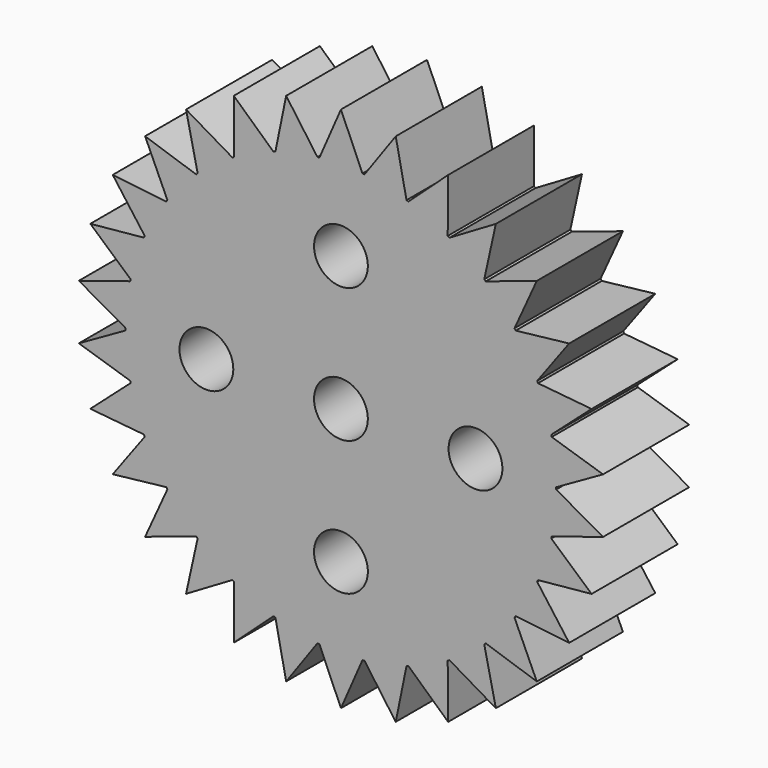
from build123d import *

# Parameters (mm, degrees)
F0_R            = 12.7
F1_DEPTH        = 3.175
F3_DEPTH        = 6.35
F3_COPIES_COUNT = 30
F4_R            = 1.5875
F5_DEPTH        = 6.35
F6_R            = 1.5875
F7_DEPTH        = 6.35
F7_COPIES_COUNT = 4


# Not quite as in the source:
# - a pattern or mirror of a feature is missing from the dataset's text; its kind, count and spacing are read off the source's solid
# - a feature names something its author has since deleted; it is built from what else it names


with BuildPart() as f1:
    # F0 (on Front) → F1 (new body, symmetric)
    with BuildSketch(Plane.XZ):
        Circle(F0_R)
    extrude(amount=F1_DEPTH, both=True)

    # F2 (on face) → F3 (join)
    with BuildSketch(Plane.XZ.offset(3.175)):
        Polygon((0, 15.5471283256), (-1.2684115066, 12.6365), (1.2684115066, 12.6365), align=None)
    f3 = extrude(amount=-F3_DEPTH)

    # F3_copies: F3 ×30 about axis
    f3_copies_axis = Axis((0, 0, 0), (0, 1, 0))
    for i in range(1, F3_COPIES_COUNT):
        add(f3.rotate(f3_copies_axis, i * 360 / F3_COPIES_COUNT))

    # F4 (on face) → F5 (cut)
    with BuildSketch(Plane.XZ.offset(3.175)):
        Circle(F4_R)
    extrude(amount=-F5_DEPTH, mode=Mode.SUBTRACT)

    # F6 (on face) → F7 (cut)
    with BuildSketch(Plane.XZ.offset(3.175)):
        with Locations((0, 7.9375)):
            Circle(F6_R)
    f7 = extrude(amount=-F7_DEPTH, mode=Mode.SUBTRACT)

    # F7_copies: F7 ×4 about axis
    f7_copies_axis = Axis((0, 0, 0), (0, 1, 0))
    for i in range(1, F7_COPIES_COUNT):
        add(f7.rotate(f7_copies_axis, i * 360 / F7_COPIES_COUNT), mode=Mode.SUBTRACT)


solid = f1.part
